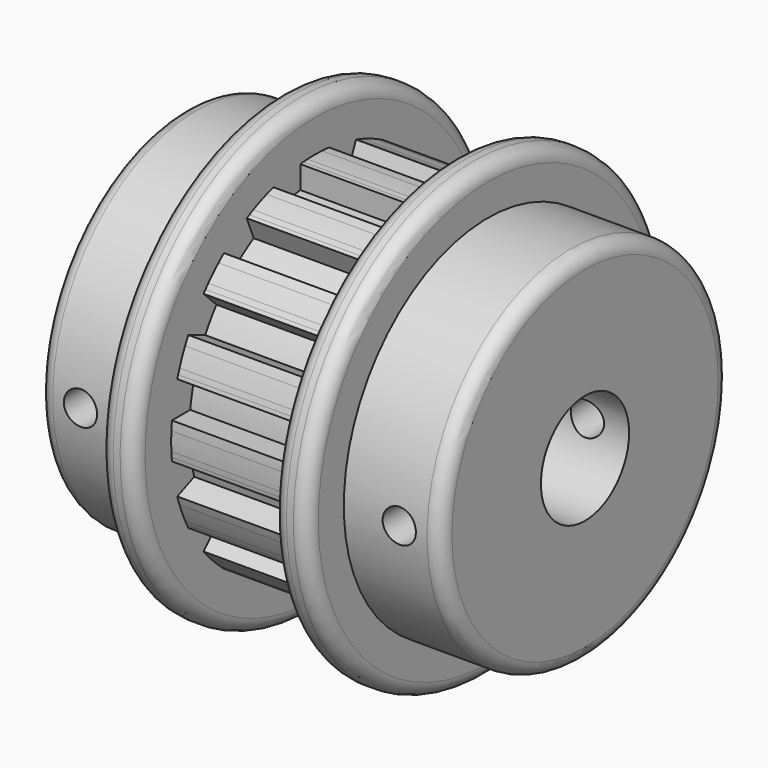
from build123d import *

# Parameters (mm, degrees)
F0_R            = 13
F0_R_2          = 3.975
F1_DEPTH        = 14.5
F2_W            = 2.5
F2_H            = 5
F4_R            = 1.2
F5_DEPTH        = 15
F2_W_2          = 10
F8_DEPTH        = 10
F8_COPIES_COUNT = 16
F9_R            = 1


# Not quite as in the source:
# - a pattern or mirror of a feature is missing from the dataset's text; its kind, count and spacing are read off the source's solid


with BuildPart() as f1:
    # F0 (on Right) → F1 (new body, symmetric)
    with BuildSketch(Plane.YZ):
        Circle(F0_R)
        Circle(F0_R_2, mode=Mode.SUBTRACT)
    extrude(amount=F1_DEPTH, both=True)

    # F2 (on Front) → F3 (revolve)
    with BuildSketch(Plane.XZ):
        with Locations((-6.25, 13.8)):
            Rectangle(F2_W, F2_H)
        with Locations((6.25, 13.8)):
            Rectangle(F2_W, F2_H)
    revolve(axis=Axis((1.1437470717, 0, 0), (1, 0, 0)))

    # F4 (on Front) → F5 (cut, symmetric)
    with BuildSketch(Plane.XZ):
        with Locations((-11.5, 0)):
            Circle(F4_R)
        with Locations((11.5, 0)):
            Circle(F4_R)
    extrude(amount=F5_DEPTH, both=True, mode=Mode.SUBTRACT)

    # F2 (on Front) → F6 (revolve, cut)
    with BuildSketch(Plane.XZ):
        with Locations((0, 13.8)):
            Rectangle(F2_W_2, F2_H)
    revolve(axis=Axis((1.1437470717, 0, 0), (1, 0, 0)), mode=Mode.SUBTRACT)

    # F7 (on face) → F8 (join)
    with BuildSketch(Plane.YZ.offset(-5)):
        with BuildLine():
            ThreePointArc((-1.3, 11.2249721603), (0, 11.3), (1.3, 11.2249721603))
            Line((1.3, 11.2249721603), (1.3, 12.8745330012))
            ThreePointArc((1.3, 12.8745330012), (0.9770986203, 12.9030569357), (0.6535840642, 12.9234835811))
            ThreePointArc((0.6535840642, 12.9234835811), (0.003296197, 12.9399995802), (-0.647, 12.923814878))
            ThreePointArc((-0.647, 12.923814878), (-0.8411950414, 12.9126291243), (-1.0352, 12.8985255343))
            ThreePointArc((-1.0352, 12.8985255343), (-1.167661625, 12.8872094082), (-1.3, 12.8745330012))
            Line((-1.3, 12.8745330012), (-1.3, 11.2249721603))
        make_face()
    f8 = extrude(amount=F8_DEPTH)

    # F8_copies: F8 ×16 about axis
    f8_copies_axis = Axis((0, 0, 0), (1, 0, 0))
    for i in range(1, F8_COPIES_COUNT):
        add(f8.rotate(f8_copies_axis, i * 360 / F8_COPIES_COUNT))

    # F9
    f9_edges = [f1.edges().sort_by_distance(p)[0] for p in [
        (-5, 0, -16.3),
        (5, 0, -16.3),
        (-14.5, -13, 0),
        (14.5, -13, 0),
        (-7.5, 0, -16.3),
        (7.5, 0, -16.3),
    ]]
    fillet(f9_edges, radius=F9_R)


solid = f1.part
